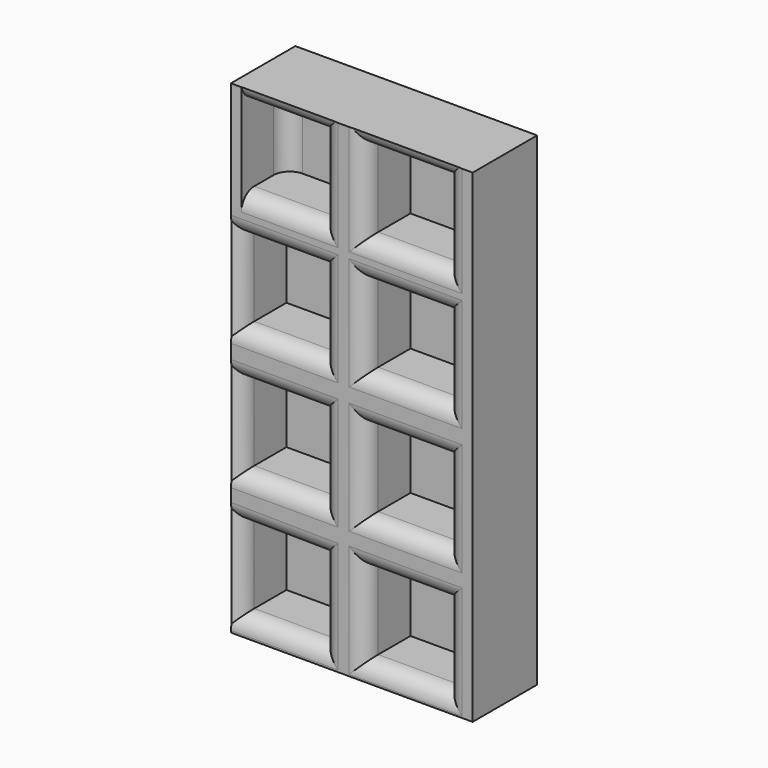
from build123d import *

# Parameters (mm, degrees)
F0_W          = 76.2
F0_H          = 152.4
F0_W_2        = 25.4
F0_H_2        = 25.4
F1_DEPTH      = 25.4
F2_DEPTH      = 7.62
F3_T1_DEPTH   = 25.4
F3_T3_DEPTH   = 25.4
F3_T5_DEPTH   = 25.4
F3_T7_DEPTH   = 25.4
F3_T9_DEPTH   = 25.4
F3_T11_DEPTH  = 25.4
F3_T13_DEPTH  = 25.4
F3_T18_DEPTH  = 50.8
F3_T23_DEPTH  = 50.8
F3_T28_DEPTH  = 50.8
F3_T33_DEPTH  = 50.8
F3_T38_DEPTH  = 50.8
F3_T43_DEPTH  = 50.8018343203
F3_T49_DEPTH  = 37.7319167972
F3_T54_DEPTH  = 38.0371819854
F3_T59_DEPTH  = 50.8
F3_T65_DEPTH  = 38.1
F3_T71_DEPTH  = 38.1
F3_T79_DEPTH  = 38.1
F3_T84_DEPTH  = 38.1
F3_T92_DEPTH  = 38.1
F3_T97_DEPTH  = 38.1
F3_T105_DEPTH = 38.1
F3_T110_DEPTH = 38.1
F3_T117_DEPTH = 38.1
F3_T122_DEPTH = 38.1
F3_T130_DEPTH = 38.1
F3_T135_DEPTH = 38.1
F3_T142_DEPTH = 38.1
F3_T147_DEPTH = 38.1
F3_T154_DEPTH = 38.1
F3_T158_DEPTH = 38.1
F3_T165_DEPTH = 38.1
F3_T171_DEPTH = 38.1
F3_T179_DEPTH = 38.1
F3_T184_DEPTH = 38.1
F3_T192_DEPTH = 38.1
F3_T197_DEPTH = 38.1
F3_T205_DEPTH = 38.1
F3_T209_DEPTH = 38.1
F3_T216_DEPTH = 38.1
F3_T220_DEPTH = 38.1
F3_T227_DEPTH = 38.1
F3_T232_DEPTH = 38.1
F3_T240_DEPTH = 38.1
F3_T244_DEPTH = 38.1
F3_T251_DEPTH = 38.1
F3_T255_DEPTH = 38.1
F3_T263_DEPTH = 38.1
F3_T267_DEPTH = 38.1
F3_T275_DEPTH = 38.1
F3_T279_DEPTH = 38.1
F3_T286_DEPTH = 38.1
F3_T290_DEPTH = 38.1
F3_T297_DEPTH = 38.1
F3_T302_DEPTH = 38.1
F3_T309_DEPTH = 38.1
F3_T314_DEPTH = 38.1
F3_T322_DEPTH = 38.1
F3_T326_DEPTH = 38.1
F3_T333_DEPTH = 38.1
F3_T338_DEPTH = 38.1
F3_T345_DEPTH = 38.1
F3_T350_DEPTH = 38.1
F3_T358_DEPTH = 38.1
F3_T362_DEPTH = 38.1
F3_T370_DEPTH = 38.0371819854
F3_T375_DEPTH = 50.8018343203
F3_T383_DEPTH = 50.8018343203
F3_T387_DEPTH = 37.7319167972
F3_T394_DEPTH = 38.1
F3_T398_DEPTH = 50.4319167972
F3_T406_DEPTH = 38.1
F3_T411_DEPTH = 50.7371819854
F3_T420_DEPTH = 38.1
F3_T425_DEPTH = 38.1


# Not quite as in the source:
# - a fillet or chamfer that OpenCascade refuses, or shapes differently, is made with other operations: its cross-section is extruded or revolved along the edge and cut away or added


with BuildPart() as f1:
    # F0 (on Front) → F1 (new body)
    with BuildSketch(Plane.XZ):
        Rectangle(F0_W, F0_H)
        Polygon((-34.8004736006, -70.5167502165), (-34.8004736006, -45.1795682311), (-9.4004736006, -45.4848334193), (-9.4004736006, -70.5167502165), align=None, mode=Mode.SUBTRACT)
        with Locations((-22.1004736006, -18.1948120378)):
            Rectangle(F0_W_2, F0_H_2, mode=Mode.SUBTRACT)
        with Locations((16.9737452313, -57.8795682311)):
            Rectangle(F0_W_2, F0_H_2, mode=Mode.SUBTRACT)
        with Locations((16.9737452313, -18.1948120378)):
            Rectangle(F0_W_2, F0_H_2, mode=Mode.SUBTRACT)
        with Locations((-22.1004736006, 21.8580199078)):
            Rectangle(F0_W_2, F0_H_2, mode=Mode.SUBTRACT)
        with Locations((-22.1004736006, 59.3430910587)):
            Rectangle(F0_W_2, F0_H_2, mode=Mode.SUBTRACT)
        with Locations((16.9737452313, 21.8580199078)):
            Rectangle(F0_W_2, F0_H_2, mode=Mode.SUBTRACT)
        with Locations((16.9737452313, 59.3430910587)):
            Rectangle(F0_W_2, F0_H_2, mode=Mode.SUBTRACT)
    extrude(amount=F1_DEPTH)

    # F0 (on Front) → F2 (join)
    with BuildSketch(Plane.XZ):
        with Locations((-22.1004736006, 59.3430910587)):
            Rectangle(F0_W_2, F0_H_2)
        with Locations((16.9737452313, 59.3430910587)):
            Rectangle(F0_W_2, F0_H_2)
        with Locations((16.9737452313, 21.8580199078)):
            Rectangle(F0_W_2, F0_H_2)
        with Locations((-22.1004736006, 21.8580199078)):
            Rectangle(F0_W_2, F0_H_2)
        with Locations((-22.1004736006, -18.1948120378)):
            Rectangle(F0_W_2, F0_H_2)
        with Locations((16.9737452313, -18.1948120378)):
            Rectangle(F0_W_2, F0_H_2)
        with Locations((16.9737452313, -57.8795682311)):
            Rectangle(F0_W_2, F0_H_2)
        Polygon((-9.4004736006, -45.4848334193), (-34.8004736006, -45.1795682311), (-34.8004736006, -70.5167502165), (-9.4004736006, -70.5167502165), align=None)
    extrude(amount=F2_DEPTH)

    # F3: fillet of radius 5.08 on 32 edges, made by hand

    # F3_s2 → F3_t1 (join)
    with BuildSketch(Plane.XY.offset(46.6430910587)):
        with BuildLine():
            ThreePointArc((-34.8004736006, -12.7), (-33.3125760491, -9.1078975516), (-29.7204736006, -7.62))
            Line((-29.7204736006, -7.62), (-34.8004736006, -7.62))
            Line((-34.8004736006, -7.62), (-34.8004736006, -12.7))
        make_face()
    extrude(amount=F3_T1_DEPTH)

    # F3_s4 → F3_t3 (cut)
    with BuildSketch(Plane.XY.offset(46.6430910587)):
        with BuildLine():
            ThreePointArc((34.7537452313, -25.4), (31.1616427829, -23.9121024484), (29.6737452313, -20.32))
            Line((29.6737452313, -20.32), (29.6737452313, -25.4))
            Line((29.6737452313, -25.4), (34.7537452313, -25.4))
        make_face()
        with BuildLine():
            ThreePointArc((-0.8062547687, -25.4), (2.7858476798, -23.9121024484), (4.2737452313, -20.32))
            Line((4.2737452313, -20.32), (4.2737452313, -25.4))
            Line((4.2737452313, -25.4), (-0.8062547687, -25.4))
        make_face()
        with BuildLine():
            ThreePointArc((-4.3204736006, -25.4), (-7.9125760491, -23.9121024484), (-9.4004736006, -20.32))
            Line((-9.4004736006, -20.32), (-9.4004736006, -25.4))
            Line((-9.4004736006, -25.4), (-4.3204736006, -25.4))
        make_face()
    extrude(amount=F3_T3_DEPTH, mode=Mode.SUBTRACT)

    # F3_s6 → F3_t5 (cut)
    with BuildSketch(Plane.YZ.offset(4.2737452313)):
        with BuildLine():
            ThreePointArc((-25.4, 77.1230910587), (-23.9121024484, 73.5309886103), (-20.32, 72.0430910587))
            Line((-20.32, 72.0430910587), (-25.4, 72.0430910587))
            Line((-25.4, 72.0430910587), (-25.4, 77.1230910587))
        make_face()
        with BuildLine():
            ThreePointArc((-25.4, 41.5630910587), (-23.9121024484, 45.1551935072), (-20.32, 46.6430910587))
            Line((-20.32, 46.6430910587), (-25.4, 46.6430910587))
            Line((-25.4, 46.6430910587), (-25.4, 41.5630910587))
        make_face()
        with BuildLine():
            ThreePointArc((-25.4, -0.4148120378), (-23.9121024484, -4.0069144862), (-20.32, -5.4948120378))
            Line((-20.32, -5.4948120378), (-25.4, -5.4948120378))
            Line((-25.4, -5.4948120378), (-25.4, -0.4148120378))
        make_face()
        with BuildLine():
            ThreePointArc((-25.4, -35.9748120378), (-23.9121024484, -32.3827095894), (-20.32, -30.8948120378))
            Line((-20.32, -30.8948120378), (-25.4, -30.8948120378))
            Line((-25.4, -30.8948120378), (-25.4, -35.9748120378))
        make_face()
        with BuildLine():
            ThreePointArc((-25.4, 39.6380199078), (-23.9121024484, 36.0459174593), (-20.32, 34.5580199078))
            Line((-20.32, 34.5580199078), (-25.4, 34.5580199078))
            Line((-25.4, 34.5580199078), (-25.4, 39.6380199078))
        make_face()
        with BuildLine():
            ThreePointArc((-25.4, -40.0995682311), (-23.9121024484, -43.6916706795), (-20.32, -45.1795682311))
            Line((-20.32, -45.1795682311), (-25.4, -45.1795682311))
            Line((-25.4, -45.1795682311), (-25.4, -40.0995682311))
        make_face()
        with BuildLine():
            ThreePointArc((-25.4, -75.6595682311), (-23.9121024484, -72.0674657827), (-20.32, -70.5795682311))
            Line((-20.32, -70.5795682311), (-25.4, -70.5795682311))
            Line((-25.4, -70.5795682311), (-25.4, -75.6595682311))
        make_face()
        with BuildLine():
            ThreePointArc((-25.4, 4.0780199078), (-23.9121024484, 7.6701223562), (-20.32, 9.1580199078))
            Line((-20.32, 9.1580199078), (-25.4, 9.1580199078))
            Line((-25.4, 9.1580199078), (-25.4, 4.0780199078))
        make_face()
    extrude(amount=F3_T5_DEPTH, mode=Mode.SUBTRACT)

    # F3_s8 → F3_t7 (cut)
    with BuildSketch(Plane.YZ.offset(-34.8004736006)):
        with BuildLine():
            ThreePointArc((-25.4, 77.1230910587), (-23.9121024484, 73.5309886103), (-20.32, 72.0430910587))
            Line((-20.32, 72.0430910587), (-25.4, 72.0430910587))
            Line((-25.4, 72.0430910587), (-25.4, 77.1230910587))
        make_face()
        with BuildLine():
            ThreePointArc((-25.4, 41.5630910587), (-23.9121024484, 45.1551935072), (-20.32, 46.6430910587))
            Line((-20.32, 46.6430910587), (-25.4, 46.6430910587))
            Line((-25.4, 46.6430910587), (-25.4, 41.5630910587))
        make_face()
        with BuildLine():
            ThreePointArc((-25.4, 39.6380199078), (-23.9121024484, 36.0459174593), (-20.32, 34.5580199078))
            Line((-20.32, 34.5580199078), (-25.4, 34.5580199078))
            Line((-25.4, 34.5580199078), (-25.4, 39.6380199078))
        make_face()
        with BuildLine():
            ThreePointArc((-25.4, 4.0780199078), (-23.9121024484, 7.6701223562), (-20.32, 9.1580199078))
            Line((-20.32, 9.1580199078), (-25.4, 9.1580199078))
            Line((-25.4, 9.1580199078), (-25.4, 4.0780199078))
        make_face()
        with BuildLine():
            ThreePointArc((-25.4, -0.4148120378), (-23.9121024484, -4.0069144862), (-20.32, -5.4948120378))
            Line((-20.32, -5.4948120378), (-25.4, -5.4948120378))
            Line((-25.4, -5.4948120378), (-25.4, -0.4148120378))
        make_face()
        with BuildLine():
            ThreePointArc((-25.4, -35.9748120378), (-23.9121024484, -32.3827095894), (-20.32, -30.8948120378))
            Line((-20.32, -30.8948120378), (-25.4, -30.8948120378))
            Line((-25.4, -30.8948120378), (-25.4, -35.9748120378))
        make_face()
        with BuildLine():
            ThreePointArc((-25.4, -75.5967502165), (-23.9121024484, -72.0046477681), (-20.32, -70.5167502165))
            Line((-20.32, -70.5167502165), (-25.4, -70.5167502165))
            Line((-25.4, -70.5167502165), (-25.4, -75.5967502165))
        make_face()
    extrude(amount=F3_T7_DEPTH, mode=Mode.SUBTRACT)

    # F3_s10 → F3_t9 (cut)
    with BuildSketch(Plane.XY.offset(9.1580199078)):
        with BuildLine():
            ThreePointArc((-4.3204736006, -25.4), (-7.9125760491, -23.9121024484), (-9.4004736006, -20.32))
            Line((-9.4004736006, -20.32), (-9.4004736006, -25.4))
            Line((-9.4004736006, -25.4), (-4.3204736006, -25.4))
        make_face()
        with BuildLine():
            ThreePointArc((-39.8804736006, -25.4), (-36.2883711522, -23.9121024484), (-34.8004736006, -20.32))
            Line((-34.8004736006, -20.32), (-34.8004736006, -25.4))
            Line((-34.8004736006, -25.4), (-39.8804736006, -25.4))
        make_face()
        with BuildLine():
            ThreePointArc((-0.8062547687, -25.4), (2.7858476798, -23.9121024484), (4.2737452313, -20.32))
            Line((4.2737452313, -20.32), (4.2737452313, -25.4))
            Line((4.2737452313, -25.4), (-0.8062547687, -25.4))
        make_face()
        with BuildLine():
            ThreePointArc((34.7537452313, -25.4), (31.1616427829, -23.9121024484), (29.6737452313, -20.32))
            Line((29.6737452313, -20.32), (29.6737452313, -25.4))
            Line((29.6737452313, -25.4), (34.7537452313, -25.4))
        make_face()
    extrude(amount=F3_T9_DEPTH, mode=Mode.SUBTRACT)

    # F3_s12 → F3_t11 (cut)
    with BuildSketch(Plane.XY.offset(-30.8948120378)):
        with BuildLine():
            ThreePointArc((-4.3204736006, -25.4), (-7.9125760491, -23.9121024484), (-9.4004736006, -20.32))
            Line((-9.4004736006, -20.32), (-9.4004736006, -25.4))
            Line((-9.4004736006, -25.4), (-4.3204736006, -25.4))
        make_face()
        with BuildLine():
            ThreePointArc((-39.8804736006, -25.4), (-36.2883711522, -23.9121024484), (-34.8004736006, -20.32))
            Line((-34.8004736006, -20.32), (-34.8004736006, -25.4))
            Line((-34.8004736006, -25.4), (-39.8804736006, -25.4))
        make_face()
        with BuildLine():
            ThreePointArc((34.7537452313, -25.4), (31.1616427829, -23.9121024484), (29.6737452313, -20.32))
            Line((29.6737452313, -20.32), (29.6737452313, -25.4))
            Line((29.6737452313, -25.4), (34.7537452313, -25.4))
        make_face()
        with BuildLine():
            ThreePointArc((-0.8062547687, -25.4), (2.7858476798, -23.9121024484), (4.2737452313, -20.32))
            Line((4.2737452313, -20.32), (4.2737452313, -25.4))
            Line((4.2737452313, -25.4), (-0.8062547687, -25.4))
        make_face()
    extrude(amount=F3_T11_DEPTH, mode=Mode.SUBTRACT)

    # F3_s14 → F3_t13 (cut)
    with BuildSketch(Plane.XY.offset(-70.5795682311)):
        with BuildLine():
            ThreePointArc((34.7537452313, -25.4), (31.1616427829, -23.9121024484), (29.6737452313, -20.32))
            Line((29.6737452313, -20.32), (29.6737452313, -25.4))
            Line((29.6737452313, -25.4), (34.7537452313, -25.4))
        make_face()
        with BuildLine():
            ThreePointArc((-0.8062547687, -25.4), (2.7858476798, -23.9121024484), (4.2737452313, -20.32))
            Line((4.2737452313, -20.32), (4.2737452313, -25.4))
            Line((4.2737452313, -25.4), (-0.8062547687, -25.4))
        make_face()
    extrude(amount=F3_T13_DEPTH, mode=Mode.SUBTRACT)


with BuildPart() as f3_tool16:
    # F3_s17 → F3_t18 (new body)
    with BuildSketch(Plane.XY.offset(84.7430910587)):
        with BuildLine():
            ThreePointArc((34.7537452313, -25.4), (31.1616427829, -23.9121024484), (29.6737452313, -20.32))
            Line((29.6737452313, -20.32), (29.6737452313, -25.4))
            Line((29.6737452313, -25.4), (34.7537452313, -25.4))
        make_face()
    extrude(amount=-F3_T18_DEPTH)

    split(bisect_by=Plane.XY.offset(34.5580199078), keep=Keep.BOTTOM)


with BuildPart() as f1_1:
    add(f1.part)

    # F3_t15: cut F3_tool16
    add(f3_tool16.part, mode=Mode.SUBTRACT)


with BuildPart() as f3_tool21:
    # F3_s22 → F3_t23 (new body)
    with BuildSketch(Plane.XY.offset(33.9430910587)):
        with BuildLine():
            ThreePointArc((-0.8062547687, -25.4), (2.7858476798, -23.9121024484), (4.2737452313, -20.32))
            Line((4.2737452313, -20.32), (4.2737452313, -25.4))
            Line((4.2737452313, -25.4), (-0.8062547687, -25.4))
        make_face()
    extrude(amount=F3_T23_DEPTH)

    split(bisect_by=Plane.XY.offset(34.5580199078), keep=Keep.BOTTOM)


with BuildPart() as f1_2:
    add(f1_1.part)

    # F3_t20: cut F3_tool21
    add(f3_tool21.part, mode=Mode.SUBTRACT)


with BuildPart() as f3_tool26:
    # F3_s27 → F3_t28 (new body)
    with BuildSketch(Plane.XY.offset(84.7430910587)):
        with BuildLine():
            ThreePointArc((-4.3204736006, -25.4), (-7.9125760491, -23.9121024484), (-9.4004736006, -20.32))
            Line((-9.4004736006, -20.32), (-9.4004736006, -25.4))
            Line((-9.4004736006, -25.4), (-4.3204736006, -25.4))
        make_face()
    extrude(amount=-F3_T28_DEPTH)

    split(bisect_by=Plane.XY.offset(34.5580199078), keep=Keep.BOTTOM)


with BuildPart() as f1_3:
    add(f1_2.part)

    # F3_t25: cut F3_tool26
    add(f3_tool26.part, mode=Mode.SUBTRACT)


with BuildPart() as f3_tool31:
    # F3_s32 → F3_t33 (new body)
    with BuildSketch(Plane.XY.offset(47.2580199078)):
        with BuildLine():
            ThreePointArc((-4.3204736006, -25.4), (-7.9125760491, -23.9121024484), (-9.4004736006, -20.32))
            Line((-9.4004736006, -20.32), (-9.4004736006, -25.4))
            Line((-9.4004736006, -25.4), (-4.3204736006, -25.4))
        make_face()
    extrude(amount=-F3_T33_DEPTH)

    split(bisect_by=Plane.XY.offset(46.6430910587), keep=Keep.TOP)


with BuildPart() as f1_4:
    add(f1_3.part)

    # F3_t30: cut F3_tool31
    add(f3_tool31.part, mode=Mode.SUBTRACT)


with BuildPart() as f3_tool36:
    # F3_s37 → F3_t38 (new body)
    with BuildSketch(Plane.XY.offset(-3.5419800922)):
        with BuildLine():
            ThreePointArc((-0.8062547687, -25.4), (2.7858476798, -23.9121024484), (4.2737452313, -20.32))
            Line((4.2737452313, -20.32), (4.2737452313, -25.4))
            Line((4.2737452313, -25.4), (-0.8062547687, -25.4))
        make_face()
    extrude(amount=F3_T38_DEPTH)

    split(bisect_by=Plane.XY.offset(46.6430910587), keep=Keep.TOP)


with BuildPart() as f1_5:
    add(f1_4.part)

    # F3_t35: cut F3_tool36
    add(f3_tool36.part, mode=Mode.SUBTRACT)


with BuildPart() as f3_tool41:
    # F3_s42 → F3_t43 (new body)
    with BuildSketch(Plane(origin=(-46.9516268134, 0, 0.5642794172), x_dir=(0, 1, 0), z_dir=(0.9999277879, 0, -0.0120174466))):
        with BuildLine():
            ThreePointArc((-25.4, -40.5145185529), (-23.9121024484, -44.1066210013), (-20.32, -45.5945185529))
            Line((-20.32, -45.5945185529), (-25.4, -45.5945185529))
            Line((-25.4, -45.5945185529), (-25.4, -40.5145185529))
        make_face()
    extrude(amount=F3_T43_DEPTH)

    split(bisect_by=Plane.YZ.offset(-34.8004736006), keep=Keep.TOP)

    split(bisect_by=Plane.YZ.offset(-9.4004736006), keep=Keep.BOTTOM)


with BuildPart() as f1_6:
    add(f1_5.part)

    # F3_t40: cut F3_tool41
    add(f3_tool41.part, mode=Mode.SUBTRACT)


with BuildPart() as f3_tool47:
    # F3_s48 → F3_t49 (new body)
    with BuildSketch(Plane.XY.offset(-32.7848334193)):
        with BuildLine():
            ThreePointArc((-4.3204736006, -25.4), (-7.9125760491, -23.9121024484), (-9.4004736006, -20.32))
            Line((-9.4004736006, -20.32), (-9.4004736006, -25.4))
            Line((-9.4004736006, -25.4), (-4.3204736006, -25.4))
        make_face()
    extrude(amount=-F3_T49_DEPTH)

    split(bisect_by=Plane(origin=(-0.5479296933, 0, -45.5912260761), x_dir=(0, 1, 0), z_dir=(-0.0120174466, 0, -0.9999277879)), keep=Keep.TOP)


with BuildPart() as f1_7:
    add(f1_6.part)

    # F3_t46: cut F3_tool47
    add(f3_tool47.part, mode=Mode.SUBTRACT)


with BuildPart() as f3_tool52:
    # F3_s53 → F3_t54 (new body)
    with BuildSketch(Plane.XY.offset(-70.5167502165)):
        with BuildLine():
            ThreePointArc((-39.8804736006, -25.4), (-36.2883711522, -23.9121024484), (-34.8004736006, -20.32))
            Line((-34.8004736006, -20.32), (-34.8004736006, -25.4))
            Line((-34.8004736006, -25.4), (-39.8804736006, -25.4))
        make_face()
    extrude(amount=F3_T54_DEPTH)

    split(bisect_by=Plane(origin=(-0.5479296933, 0, -45.5912260761), x_dir=(0, 1, 0), z_dir=(-0.0120174466, 0, -0.9999277879)), keep=Keep.TOP)


with BuildPart() as f1_8:
    add(f1_7.part)

    # F3_t51: cut F3_tool52
    add(f3_tool52.part, mode=Mode.SUBTRACT)


with BuildPart() as f3_tool57:
    # F3_s58 → F3_t59 (new body)
    with BuildSketch(Plane.XY.offset(47.2580199078)):
        with BuildLine():
            ThreePointArc((34.7537452313, -25.4), (31.1616427829, -23.9121024484), (29.6737452313, -20.32))
            Line((29.6737452313, -20.32), (29.6737452313, -25.4))
            Line((29.6737452313, -25.4), (34.7537452313, -25.4))
        make_face()
    extrude(amount=-F3_T59_DEPTH)

    split(bisect_by=Plane.XY.offset(46.6430910587), keep=Keep.TOP)


with BuildPart() as f1_9:
    add(f1_8.part)

    # F3_t56: cut F3_tool57
    add(f3_tool57.part, mode=Mode.SUBTRACT)


with BuildPart() as f3_tool63:
    # F3_s64 → F3_t65 (new body)
    with BuildSketch(Plane.YZ.offset(4.2737452313)):
        with BuildLine():
            ThreePointArc((-25.4, 77.1230910587), (-23.9121024484, 73.5309886103), (-20.32, 72.0430910587))
            Line((-20.32, 72.0430910587), (-25.4, 72.0430910587))
            Line((-25.4, 72.0430910587), (-25.4, 77.1230910587))
        make_face()
    extrude(amount=F3_T65_DEPTH)

    split(bisect_by=Plane.YZ.offset(38.1), keep=Keep.BOTTOM)

    split(bisect_by=Plane.XY.offset(76.2), keep=Keep.BOTTOM)

    split(bisect_by=Plane.YZ.offset(29.6737452313), keep=Keep.TOP)


with BuildPart() as f3_tool69:
    # F3_s70 → F3_t71 (new body)
    with BuildSketch(Plane.XY.offset(84.7430910587)):
        with BuildLine():
            ThreePointArc((34.7537452313, -25.4), (31.1616427829, -23.9121024484), (29.6737452313, -20.32))
            Line((29.6737452313, -20.32), (29.6737452313, -25.4))
            Line((29.6737452313, -25.4), (34.7537452313, -25.4))
        make_face()
    extrude(amount=-F3_T71_DEPTH)

    split(bisect_by=Plane.XY.offset(76.2), keep=Keep.BOTTOM)

    split(bisect_by=Plane.XY.offset(72.0430910587), keep=Keep.TOP)


with BuildPart() as f3_tool63_1:
    add(f3_tool63.part)

    # F3_t74: intersect F3_tool69
    add(f3_tool69.part, mode=Mode.INTERSECT)


with BuildPart() as f1_10:
    add(f1_9.part)

    # F3_t61: cut F3_tool63
    add(f3_tool63_1.part, mode=Mode.SUBTRACT)


with BuildPart() as f3_tool77:
    # F3_s78 → F3_t79 (new body)
    with BuildSketch(Plane.XY.offset(72.0430910587)):
        with BuildLine():
            ThreePointArc((34.7537452313, -25.4), (31.1616427829, -23.9121024484), (29.6737452313, -20.32))
            Line((29.6737452313, -20.32), (29.6737452313, -25.4))
            Line((29.6737452313, -25.4), (34.7537452313, -25.4))
        make_face()
    extrude(amount=-F3_T79_DEPTH)

    split(bisect_by=Plane.XY.offset(34.5580199078), keep=Keep.TOP)

    split(bisect_by=Plane.XY.offset(46.6430910587), keep=Keep.BOTTOM)


with BuildPart() as f3_tool82:
    # F3_s83 → F3_t84 (new body)
    with BuildSketch(Plane.YZ.offset(42.3737452313)):
        with BuildLine():
            ThreePointArc((-25.4, 41.5630910587), (-23.9121024484, 45.1551935072), (-20.32, 46.6430910587))
            Line((-20.32, 46.6430910587), (-25.4, 46.6430910587))
            Line((-25.4, 46.6430910587), (-25.4, 41.5630910587))
        make_face()
    extrude(amount=-F3_T84_DEPTH)

    split(bisect_by=Plane.YZ.offset(38.1), keep=Keep.BOTTOM)

    split(bisect_by=Plane.YZ.offset(29.6737452313), keep=Keep.TOP)


with BuildPart() as f3_tool77_1:
    add(f3_tool77.part)

    # F3_t87: intersect F3_tool82
    add(f3_tool82.part, mode=Mode.INTERSECT)


with BuildPart() as f1_11:
    add(f1_10.part)

    # F3_t75: cut F3_tool77
    add(f3_tool77_1.part, mode=Mode.SUBTRACT)


with BuildPart() as f3_tool90:
    # F3_s91 → F3_t92 (new body)
    with BuildSketch(Plane.XY.offset(46.6430910587)):
        with BuildLine():
            ThreePointArc((-0.8062547687, -25.4), (2.7858476798, -23.9121024484), (4.2737452313, -20.32))
            Line((4.2737452313, -20.32), (4.2737452313, -25.4))
            Line((4.2737452313, -25.4), (-0.8062547687, -25.4))
        make_face()
    extrude(amount=F3_T92_DEPTH)

    split(bisect_by=Plane.XY.offset(76.2), keep=Keep.BOTTOM)

    split(bisect_by=Plane.XY.offset(72.0430910587), keep=Keep.TOP)


with BuildPart() as f3_tool95:
    # F3_s96 → F3_t97 (new body)
    with BuildSketch(Plane.YZ.offset(-8.4262547687)):
        with BuildLine():
            ThreePointArc((-25.4, 77.1230910587), (-23.9121024484, 73.5309886103), (-20.32, 72.0430910587))
            Line((-20.32, 72.0430910587), (-25.4, 72.0430910587))
            Line((-25.4, 72.0430910587), (-25.4, 77.1230910587))
        make_face()
    extrude(amount=F3_T97_DEPTH)

    split(bisect_by=Plane.XY.offset(76.2), keep=Keep.BOTTOM)

    split(bisect_by=Plane.YZ.offset(4.2737452313), keep=Keep.BOTTOM)


with BuildPart() as f3_tool90_1:
    add(f3_tool90.part)

    # F3_t100: intersect F3_tool95
    add(f3_tool95.part, mode=Mode.INTERSECT)


with BuildPart() as f1_12:
    add(f1_11.part)

    # F3_t88: cut F3_tool90
    add(f3_tool90_1.part, mode=Mode.SUBTRACT)


with BuildPart() as f3_tool103:
    # F3_s104 → F3_t105 (new body)
    with BuildSketch(Plane.XY.offset(33.9430910587)):
        with BuildLine():
            ThreePointArc((-0.8062547687, -25.4), (2.7858476798, -23.9121024484), (4.2737452313, -20.32))
            Line((4.2737452313, -20.32), (4.2737452313, -25.4))
            Line((4.2737452313, -25.4), (-0.8062547687, -25.4))
        make_face()
    extrude(amount=F3_T105_DEPTH)

    split(bisect_by=Plane.XY.offset(34.5580199078), keep=Keep.TOP)

    split(bisect_by=Plane.XY.offset(46.6430910587), keep=Keep.BOTTOM)


with BuildPart() as f3_tool108:
    # F3_s109 → F3_t110 (new body)
    with BuildSketch(Plane.YZ.offset(29.6737452313)):
        with BuildLine():
            ThreePointArc((-25.4, 41.5630910587), (-23.9121024484, 45.1551935072), (-20.32, 46.6430910587))
            Line((-20.32, 46.6430910587), (-25.4, 46.6430910587))
            Line((-25.4, 46.6430910587), (-25.4, 41.5630910587))
        make_face()
    extrude(amount=-F3_T110_DEPTH)

    split(bisect_by=Plane.YZ.offset(4.2737452313), keep=Keep.BOTTOM)


with BuildPart() as f3_tool103_1:
    add(f3_tool103.part)

    # F3_t112: intersect F3_tool108
    add(f3_tool108.part, mode=Mode.INTERSECT)


with BuildPart() as f1_13:
    add(f1_12.part)

    # F3_t101: cut F3_tool103
    add(f3_tool103_1.part, mode=Mode.SUBTRACT)


with BuildPart() as f3_tool115:
    # F3_s116 → F3_t117 (new body)
    with BuildSketch(Plane.YZ.offset(-34.8004736006)):
        with BuildLine():
            ThreePointArc((-25.4, 77.1230910587), (-23.9121024484, 73.5309886103), (-20.32, 72.0430910587))
            Line((-20.32, 72.0430910587), (-25.4, 72.0430910587))
            Line((-25.4, 72.0430910587), (-25.4, 77.1230910587))
        make_face()
    extrude(amount=F3_T117_DEPTH)

    split(bisect_by=Plane.XY.offset(76.2), keep=Keep.BOTTOM)

    split(bisect_by=Plane.YZ.offset(-9.4004736006), keep=Keep.TOP)


with BuildPart() as f3_tool120:
    # F3_s121 → F3_t122 (new body)
    with BuildSketch(Plane.XY.offset(84.7430910587)):
        with BuildLine():
            ThreePointArc((-4.3204736006, -25.4), (-7.9125760491, -23.9121024484), (-9.4004736006, -20.32))
            Line((-9.4004736006, -20.32), (-9.4004736006, -25.4))
            Line((-9.4004736006, -25.4), (-4.3204736006, -25.4))
        make_face()
    extrude(amount=-F3_T122_DEPTH)

    split(bisect_by=Plane.XY.offset(76.2), keep=Keep.BOTTOM)

    split(bisect_by=Plane.XY.offset(72.0430910587), keep=Keep.TOP)


with BuildPart() as f3_tool115_1:
    add(f3_tool115.part)

    # F3_t125: intersect F3_tool120
    add(f3_tool120.part, mode=Mode.INTERSECT)


with BuildPart() as f1_14:
    add(f1_13.part)

    # F3_t113: cut F3_tool115
    add(f3_tool115_1.part, mode=Mode.SUBTRACT)


with BuildPart() as f3_tool128:
    # F3_s129 → F3_t130 (new body)
    with BuildSketch(Plane.XY.offset(72.0430910587)):
        with BuildLine():
            ThreePointArc((-4.3204736006, -25.4), (-7.9125760491, -23.9121024484), (-9.4004736006, -20.32))
            Line((-9.4004736006, -20.32), (-9.4004736006, -25.4))
            Line((-9.4004736006, -25.4), (-4.3204736006, -25.4))
        make_face()
    extrude(amount=-F3_T130_DEPTH)

    split(bisect_by=Plane.XY.offset(34.5580199078), keep=Keep.TOP)

    split(bisect_by=Plane.XY.offset(46.6430910587), keep=Keep.BOTTOM)


with BuildPart() as f3_tool133:
    # F3_s134 → F3_t135 (new body)
    with BuildSketch(Plane.YZ.offset(3.2995263994)):
        with BuildLine():
            ThreePointArc((-25.4, 41.5630910587), (-23.9121024484, 45.1551935072), (-20.32, 46.6430910587))
            Line((-20.32, 46.6430910587), (-25.4, 46.6430910587))
            Line((-25.4, 46.6430910587), (-25.4, 41.5630910587))
        make_face()
    extrude(amount=-F3_T135_DEPTH)

    split(bisect_by=Plane.YZ.offset(-9.4004736006), keep=Keep.TOP)


with BuildPart() as f3_tool128_1:
    add(f3_tool128.part)

    # F3_t137: intersect F3_tool133
    add(f3_tool133.part, mode=Mode.INTERSECT)


with BuildPart() as f1_15:
    add(f1_14.part)

    # F3_t126: cut F3_tool128
    add(f3_tool128_1.part, mode=Mode.SUBTRACT)


with BuildPart() as f3_tool140:
    # F3_s141 → F3_t142 (new body)
    with BuildSketch(Plane.XY.offset(47.2580199078)):
        with BuildLine():
            ThreePointArc((-4.3204736006, -25.4), (-7.9125760491, -23.9121024484), (-9.4004736006, -20.32))
            Line((-9.4004736006, -20.32), (-9.4004736006, -25.4))
            Line((-9.4004736006, -25.4), (-4.3204736006, -25.4))
        make_face()
    extrude(amount=-F3_T142_DEPTH)

    split(bisect_by=Plane.XY.offset(34.5580199078), keep=Keep.TOP)

    split(bisect_by=Plane.XY.offset(46.6430910587), keep=Keep.BOTTOM)


with BuildPart() as f3_tool145:
    # F3_s146 → F3_t147 (new body)
    with BuildSketch(Plane.YZ.offset(-34.8004736006)):
        with BuildLine():
            ThreePointArc((-25.4, 39.6380199078), (-23.9121024484, 36.0459174593), (-20.32, 34.5580199078))
            Line((-20.32, 34.5580199078), (-25.4, 34.5580199078))
            Line((-25.4, 34.5580199078), (-25.4, 39.6380199078))
        make_face()
    extrude(amount=F3_T147_DEPTH)

    split(bisect_by=Plane.YZ.offset(-9.4004736006), keep=Keep.TOP)


with BuildPart() as f3_tool140_1:
    add(f3_tool140.part)

    # F3_t149: intersect F3_tool145
    add(f3_tool145.part, mode=Mode.INTERSECT)


with BuildPart() as f1_16:
    add(f1_15.part)

    # F3_t138: cut F3_tool140
    add(f3_tool140_1.part, mode=Mode.SUBTRACT)


with BuildPart() as f3_tool152:
    # F3_s153 → F3_t154 (new body)
    with BuildSketch(Plane.XY.offset(34.5580199078)):
        with BuildLine():
            ThreePointArc((-4.3204736006, -25.4), (-7.9125760491, -23.9121024484), (-9.4004736006, -20.32))
            Line((-9.4004736006, -20.32), (-9.4004736006, -25.4))
            Line((-9.4004736006, -25.4), (-4.3204736006, -25.4))
        make_face()
    extrude(amount=-F3_T154_DEPTH)

    split(bisect_by=Plane.XY.offset(9.1580199078), keep=Keep.BOTTOM)


with BuildPart() as f3_tool156:
    # F3_s157 → F3_t158 (new body)
    with BuildSketch(Plane.YZ.offset(3.2995263994)):
        with BuildLine():
            ThreePointArc((-25.4, 4.0780199078), (-23.9121024484, 7.6701223562), (-20.32, 9.1580199078))
            Line((-20.32, 9.1580199078), (-25.4, 9.1580199078))
            Line((-25.4, 9.1580199078), (-25.4, 4.0780199078))
        make_face()
    extrude(amount=-F3_T158_DEPTH)

    split(bisect_by=Plane.YZ.offset(-9.4004736006), keep=Keep.TOP)


with BuildPart() as f3_tool152_1:
    add(f3_tool152.part)

    # F3_t160: intersect F3_tool156
    add(f3_tool156.part, mode=Mode.INTERSECT)


with BuildPart() as f1_17:
    add(f1_16.part)

    # F3_t150: cut F3_tool152
    add(f3_tool152_1.part, mode=Mode.SUBTRACT)


with BuildPart() as f3_tool163:
    # F3_s164 → F3_t165 (new body)
    with BuildSketch(Plane.XY.offset(9.1580199078)):
        with BuildLine():
            ThreePointArc((-39.8804736006, -25.4), (-36.2883711522, -23.9121024484), (-34.8004736006, -20.32))
            Line((-34.8004736006, -20.32), (-34.8004736006, -25.4))
            Line((-34.8004736006, -25.4), (-39.8804736006, -25.4))
        make_face()
    extrude(amount=F3_T165_DEPTH)

    split(bisect_by=Plane.YZ.offset(-38.1), keep=Keep.TOP)

    split(bisect_by=Plane.XY.offset(34.5580199078), keep=Keep.TOP)

    split(bisect_by=Plane.XY.offset(46.6430910587), keep=Keep.BOTTOM)


with BuildPart() as f3_tool169:
    # F3_s170 → F3_t171 (new body)
    with BuildSketch(Plane.YZ.offset(-47.5004736006)):
        with BuildLine():
            ThreePointArc((-25.4, 39.6380199078), (-23.9121024484, 36.0459174593), (-20.32, 34.5580199078))
            Line((-20.32, 34.5580199078), (-25.4, 34.5580199078))
            Line((-25.4, 34.5580199078), (-25.4, 39.6380199078))
        make_face()
    extrude(amount=F3_T171_DEPTH)

    split(bisect_by=Plane.YZ.offset(-38.1), keep=Keep.TOP)

    split(bisect_by=Plane.YZ.offset(-34.8004736006), keep=Keep.BOTTOM)


with BuildPart() as f3_tool163_1:
    add(f3_tool163.part)

    # F3_t174: intersect F3_tool169
    add(f3_tool169.part, mode=Mode.INTERSECT)


with BuildPart() as f1_18:
    add(f1_17.part)

    # F3_t161: cut F3_tool163
    add(f3_tool163_1.part, mode=Mode.SUBTRACT)


with BuildPart() as f3_tool177:
    # F3_s178 → F3_t179 (new body)
    with BuildSketch(Plane.YZ.offset(-9.4004736006)):
        with BuildLine():
            ThreePointArc((-25.4, 4.0780199078), (-23.9121024484, 7.6701223562), (-20.32, 9.1580199078))
            Line((-20.32, 9.1580199078), (-25.4, 9.1580199078))
            Line((-25.4, 9.1580199078), (-25.4, 4.0780199078))
        make_face()
    extrude(amount=-F3_T179_DEPTH)

    split(bisect_by=Plane.YZ.offset(-38.1), keep=Keep.TOP)

    split(bisect_by=Plane.YZ.offset(-34.8004736006), keep=Keep.BOTTOM)


with BuildPart() as f3_tool182:
    # F3_s183 → F3_t184 (new body)
    with BuildSketch(Plane.XY.offset(-3.5419800922)):
        with BuildLine():
            ThreePointArc((-39.8804736006, -25.4), (-36.2883711522, -23.9121024484), (-34.8004736006, -20.32))
            Line((-34.8004736006, -20.32), (-34.8004736006, -25.4))
            Line((-34.8004736006, -25.4), (-39.8804736006, -25.4))
        make_face()
    extrude(amount=F3_T184_DEPTH)

    split(bisect_by=Plane.YZ.offset(-38.1), keep=Keep.TOP)

    split(bisect_by=Plane.XY.offset(9.1580199078), keep=Keep.BOTTOM)


with BuildPart() as f3_tool177_1:
    add(f3_tool177.part)

    # F3_t187: intersect F3_tool182
    add(f3_tool182.part, mode=Mode.INTERSECT)


with BuildPart() as f1_19:
    add(f1_18.part)

    # F3_t175: cut F3_tool177
    add(f3_tool177_1.part, mode=Mode.SUBTRACT)


with BuildPart() as f3_tool190:
    # F3_s191 → F3_t192 (new body)
    with BuildSketch(Plane.XY.offset(-30.8948120378)):
        with BuildLine():
            ThreePointArc((-39.8804736006, -25.4), (-36.2883711522, -23.9121024484), (-34.8004736006, -20.32))
            Line((-34.8004736006, -20.32), (-34.8004736006, -25.4))
            Line((-34.8004736006, -25.4), (-39.8804736006, -25.4))
        make_face()
    extrude(amount=F3_T192_DEPTH)

    split(bisect_by=Plane.YZ.offset(-38.1), keep=Keep.TOP)

    split(bisect_by=Plane.XY.offset(-5.4948120378), keep=Keep.TOP)


with BuildPart() as f3_tool195:
    # F3_s196 → F3_t197 (new body)
    with BuildSketch(Plane.YZ.offset(-47.5004736006)):
        with BuildLine():
            ThreePointArc((-25.4, -0.4148120378), (-23.9121024484, -4.0069144862), (-20.32, -5.4948120378))
            Line((-20.32, -5.4948120378), (-25.4, -5.4948120378))
            Line((-25.4, -5.4948120378), (-25.4, -0.4148120378))
        make_face()
    extrude(amount=F3_T197_DEPTH)

    split(bisect_by=Plane.YZ.offset(-38.1), keep=Keep.TOP)

    split(bisect_by=Plane.YZ.offset(-34.8004736006), keep=Keep.BOTTOM)


with BuildPart() as f3_tool190_1:
    add(f3_tool190.part)

    # F3_t200: intersect F3_tool195
    add(f3_tool195.part, mode=Mode.INTERSECT)


with BuildPart() as f1_20:
    add(f1_19.part)

    # F3_t188: cut F3_tool190
    add(f3_tool190_1.part, mode=Mode.SUBTRACT)


with BuildPart() as f3_tool203:
    # F3_s204 → F3_t205 (new body)
    with BuildSketch(Plane.YZ.offset(-34.8004736006)):
        with BuildLine():
            ThreePointArc((-25.4, -0.4148120378), (-23.9121024484, -4.0069144862), (-20.32, -5.4948120378))
            Line((-20.32, -5.4948120378), (-25.4, -5.4948120378))
            Line((-25.4, -5.4948120378), (-25.4, -0.4148120378))
        make_face()
    extrude(amount=F3_T205_DEPTH)

    split(bisect_by=Plane.YZ.offset(-9.4004736006), keep=Keep.TOP)


with BuildPart() as f3_tool207:
    # F3_s208 → F3_t209 (new body)
    with BuildSketch(Plane.XY.offset(7.2051879622)):
        with BuildLine():
            ThreePointArc((-4.3204736006, -25.4), (-7.9125760491, -23.9121024484), (-9.4004736006, -20.32))
            Line((-9.4004736006, -20.32), (-9.4004736006, -25.4))
            Line((-9.4004736006, -25.4), (-4.3204736006, -25.4))
        make_face()
    extrude(amount=-F3_T209_DEPTH)

    split(bisect_by=Plane.XY.offset(-5.4948120378), keep=Keep.TOP)


with BuildPart() as f3_tool203_1:
    add(f3_tool203.part)

    # F3_t211: intersect F3_tool207
    add(f3_tool207.part, mode=Mode.INTERSECT)


with BuildPart() as f1_21:
    add(f1_20.part)

    # F3_t201: cut F3_tool203
    add(f3_tool203_1.part, mode=Mode.SUBTRACT)


with BuildPart() as f3_tool214:
    # F3_s215 → F3_t216 (new body)
    with BuildSketch(Plane.XY.offset(-5.4948120378)):
        with BuildLine():
            ThreePointArc((-4.3204736006, -25.4), (-7.9125760491, -23.9121024484), (-9.4004736006, -20.32))
            Line((-9.4004736006, -20.32), (-9.4004736006, -25.4))
            Line((-9.4004736006, -25.4), (-4.3204736006, -25.4))
        make_face()
    extrude(amount=-F3_T216_DEPTH)

    split(bisect_by=Plane.XY.offset(-30.8948120378), keep=Keep.BOTTOM)


with BuildPart() as f3_tool218:
    # F3_s219 → F3_t220 (new body)
    with BuildSketch(Plane.YZ.offset(3.2995263994)):
        with BuildLine():
            ThreePointArc((-25.4, -35.9748120378), (-23.9121024484, -32.3827095894), (-20.32, -30.8948120378))
            Line((-20.32, -30.8948120378), (-25.4, -30.8948120378))
            Line((-25.4, -30.8948120378), (-25.4, -35.9748120378))
        make_face()
    extrude(amount=-F3_T220_DEPTH)

    split(bisect_by=Plane.YZ.offset(-9.4004736006), keep=Keep.TOP)


with BuildPart() as f3_tool214_1:
    add(f3_tool214.part)

    # F3_t222: intersect F3_tool218
    add(f3_tool218.part, mode=Mode.INTERSECT)


with BuildPart() as f1_22:
    add(f1_21.part)

    # F3_t212: cut F3_tool214
    add(f3_tool214_1.part, mode=Mode.SUBTRACT)


with BuildPart() as f3_tool225:
    # F3_s226 → F3_t227 (new body)
    with BuildSketch(Plane.XY.offset(-43.5948120378)):
        with BuildLine():
            ThreePointArc((-39.8804736006, -25.4), (-36.2883711522, -23.9121024484), (-34.8004736006, -20.32))
            Line((-34.8004736006, -20.32), (-34.8004736006, -25.4))
            Line((-34.8004736006, -25.4), (-39.8804736006, -25.4))
        make_face()
    extrude(amount=F3_T227_DEPTH)

    split(bisect_by=Plane.YZ.offset(-38.1), keep=Keep.TOP)

    split(bisect_by=Plane.XY.offset(-30.8948120378), keep=Keep.BOTTOM)


with BuildPart() as f3_tool230:
    # F3_s231 → F3_t232 (new body)
    with BuildSketch(Plane.YZ.offset(-9.4004736006)):
        with BuildLine():
            ThreePointArc((-25.4, -35.9748120378), (-23.9121024484, -32.3827095894), (-20.32, -30.8948120378))
            Line((-20.32, -30.8948120378), (-25.4, -30.8948120378))
            Line((-25.4, -30.8948120378), (-25.4, -35.9748120378))
        make_face()
    extrude(amount=-F3_T232_DEPTH)

    split(bisect_by=Plane.YZ.offset(-38.1), keep=Keep.TOP)

    split(bisect_by=Plane.YZ.offset(-34.8004736006), keep=Keep.BOTTOM)


with BuildPart() as f3_tool225_1:
    add(f3_tool225.part)

    # F3_t235: intersect F3_tool230
    add(f3_tool230.part, mode=Mode.INTERSECT)


with BuildPart() as f1_23:
    add(f1_22.part)

    # F3_t223: cut F3_tool225
    add(f3_tool225_1.part, mode=Mode.SUBTRACT)


with BuildPart() as f3_tool238:
    # F3_s239 → F3_t240 (new body)
    with BuildSketch(Plane.XY.offset(-30.8948120378)):
        with BuildLine():
            ThreePointArc((-0.8062547687, -25.4), (2.7858476798, -23.9121024484), (4.2737452313, -20.32))
            Line((4.2737452313, -20.32), (4.2737452313, -25.4))
            Line((4.2737452313, -25.4), (-0.8062547687, -25.4))
        make_face()
    extrude(amount=F3_T240_DEPTH)

    split(bisect_by=Plane.XY.offset(-5.4948120378), keep=Keep.TOP)


with BuildPart() as f3_tool242:
    # F3_s243 → F3_t244 (new body)
    with BuildSketch(Plane.YZ.offset(-8.4262547687)):
        with BuildLine():
            ThreePointArc((-25.4, -0.4148120378), (-23.9121024484, -4.0069144862), (-20.32, -5.4948120378))
            Line((-20.32, -5.4948120378), (-25.4, -5.4948120378))
            Line((-25.4, -5.4948120378), (-25.4, -0.4148120378))
        make_face()
    extrude(amount=F3_T244_DEPTH)

    split(bisect_by=Plane.YZ.offset(4.2737452313), keep=Keep.BOTTOM)


with BuildPart() as f3_tool238_1:
    add(f3_tool238.part)

    # F3_t246: intersect F3_tool242
    add(f3_tool242.part, mode=Mode.INTERSECT)


with BuildPart() as f1_24:
    add(f1_23.part)

    # F3_t236: cut F3_tool238
    add(f3_tool238_1.part, mode=Mode.SUBTRACT)


with BuildPart() as f3_tool249:
    # F3_s250 → F3_t251 (new body)
    with BuildSketch(Plane.XY.offset(7.2051879622)):
        with BuildLine():
            ThreePointArc((34.7537452313, -25.4), (31.1616427829, -23.9121024484), (29.6737452313, -20.32))
            Line((29.6737452313, -20.32), (29.6737452313, -25.4))
            Line((29.6737452313, -25.4), (34.7537452313, -25.4))
        make_face()
    extrude(amount=-F3_T251_DEPTH)

    split(bisect_by=Plane.XY.offset(-5.4948120378), keep=Keep.TOP)


with BuildPart() as f3_tool253:
    # F3_s254 → F3_t255 (new body)
    with BuildSketch(Plane.YZ.offset(4.2737452313)):
        with BuildLine():
            ThreePointArc((-25.4, -0.4148120378), (-23.9121024484, -4.0069144862), (-20.32, -5.4948120378))
            Line((-20.32, -5.4948120378), (-25.4, -5.4948120378))
            Line((-25.4, -5.4948120378), (-25.4, -0.4148120378))
        make_face()
    extrude(amount=F3_T255_DEPTH)

    split(bisect_by=Plane.YZ.offset(38.1), keep=Keep.BOTTOM)

    split(bisect_by=Plane.YZ.offset(29.6737452313), keep=Keep.TOP)


with BuildPart() as f3_tool249_1:
    add(f3_tool249.part)

    # F3_t258: intersect F3_tool253
    add(f3_tool253.part, mode=Mode.INTERSECT)


with BuildPart() as f1_25:
    add(f1_24.part)

    # F3_t247: cut F3_tool249
    add(f3_tool249_1.part, mode=Mode.SUBTRACT)


with BuildPart() as f3_tool261:
    # F3_s262 → F3_t263 (new body)
    with BuildSketch(Plane.XY.offset(-5.4948120378)):
        with BuildLine():
            ThreePointArc((34.7537452313, -25.4), (31.1616427829, -23.9121024484), (29.6737452313, -20.32))
            Line((29.6737452313, -20.32), (29.6737452313, -25.4))
            Line((29.6737452313, -25.4), (34.7537452313, -25.4))
        make_face()
    extrude(amount=-F3_T263_DEPTH)

    split(bisect_by=Plane.XY.offset(-30.8948120378), keep=Keep.BOTTOM)


with BuildPart() as f3_tool265:
    # F3_s266 → F3_t267 (new body)
    with BuildSketch(Plane.YZ.offset(42.3737452313)):
        with BuildLine():
            ThreePointArc((-25.4, -35.9748120378), (-23.9121024484, -32.3827095894), (-20.32, -30.8948120378))
            Line((-20.32, -30.8948120378), (-25.4, -30.8948120378))
            Line((-25.4, -30.8948120378), (-25.4, -35.9748120378))
        make_face()
    extrude(amount=-F3_T267_DEPTH)

    split(bisect_by=Plane.YZ.offset(38.1), keep=Keep.BOTTOM)

    split(bisect_by=Plane.YZ.offset(29.6737452313), keep=Keep.TOP)


with BuildPart() as f3_tool261_1:
    add(f3_tool261.part)

    # F3_t270: intersect F3_tool265
    add(f3_tool265.part, mode=Mode.INTERSECT)


with BuildPart() as f1_26:
    add(f1_25.part)

    # F3_t259: cut F3_tool261
    add(f3_tool261_1.part, mode=Mode.SUBTRACT)


with BuildPart() as f3_tool273:
    # F3_s274 → F3_t275 (new body)
    with BuildSketch(Plane.YZ.offset(29.6737452313)):
        with BuildLine():
            ThreePointArc((-25.4, -35.9748120378), (-23.9121024484, -32.3827095894), (-20.32, -30.8948120378))
            Line((-20.32, -30.8948120378), (-25.4, -30.8948120378))
            Line((-25.4, -30.8948120378), (-25.4, -35.9748120378))
        make_face()
    extrude(amount=-F3_T275_DEPTH)

    split(bisect_by=Plane.YZ.offset(4.2737452313), keep=Keep.BOTTOM)


with BuildPart() as f3_tool277:
    # F3_s278 → F3_t279 (new body)
    with BuildSketch(Plane.XY.offset(-43.5948120378)):
        with BuildLine():
            ThreePointArc((-0.8062547687, -25.4), (2.7858476798, -23.9121024484), (4.2737452313, -20.32))
            Line((4.2737452313, -20.32), (4.2737452313, -25.4))
            Line((4.2737452313, -25.4), (-0.8062547687, -25.4))
        make_face()
    extrude(amount=F3_T279_DEPTH)

    split(bisect_by=Plane.XY.offset(-30.8948120378), keep=Keep.BOTTOM)


with BuildPart() as f3_tool273_1:
    add(f3_tool273.part)

    # F3_t281: intersect F3_tool277
    add(f3_tool277.part, mode=Mode.INTERSECT)


with BuildPart() as f1_27:
    add(f1_26.part)

    # F3_t271: cut F3_tool273
    add(f3_tool273_1.part, mode=Mode.SUBTRACT)


with BuildPart() as f3_tool284:
    # F3_s285 → F3_t286 (new body)
    with BuildSketch(Plane.YZ.offset(29.6737452313)):
        with BuildLine():
            ThreePointArc((-25.4, 4.0780199078), (-23.9121024484, 7.6701223562), (-20.32, 9.1580199078))
            Line((-20.32, 9.1580199078), (-25.4, 9.1580199078))
            Line((-25.4, 9.1580199078), (-25.4, 4.0780199078))
        make_face()
    extrude(amount=-F3_T286_DEPTH)

    split(bisect_by=Plane.YZ.offset(4.2737452313), keep=Keep.BOTTOM)


with BuildPart() as f3_tool288:
    # F3_s289 → F3_t290 (new body)
    with BuildSketch(Plane.XY.offset(-3.5419800922)):
        with BuildLine():
            ThreePointArc((-0.8062547687, -25.4), (2.7858476798, -23.9121024484), (4.2737452313, -20.32))
            Line((4.2737452313, -20.32), (4.2737452313, -25.4))
            Line((4.2737452313, -25.4), (-0.8062547687, -25.4))
        make_face()
    extrude(amount=F3_T290_DEPTH)

    split(bisect_by=Plane.XY.offset(9.1580199078), keep=Keep.BOTTOM)


with BuildPart() as f3_tool284_1:
    add(f3_tool284.part)

    # F3_t292: intersect F3_tool288
    add(f3_tool288.part, mode=Mode.INTERSECT)


with BuildPart() as f1_28:
    add(f1_27.part)

    # F3_t282: cut F3_tool284
    add(f3_tool284_1.part, mode=Mode.SUBTRACT)


with BuildPart() as f3_tool295:
    # F3_s296 → F3_t297 (new body)
    with BuildSketch(Plane.XY.offset(9.1580199078)):
        with BuildLine():
            ThreePointArc((-0.8062547687, -25.4), (2.7858476798, -23.9121024484), (4.2737452313, -20.32))
            Line((4.2737452313, -20.32), (4.2737452313, -25.4))
            Line((4.2737452313, -25.4), (-0.8062547687, -25.4))
        make_face()
    extrude(amount=F3_T297_DEPTH)

    split(bisect_by=Plane.XY.offset(34.5580199078), keep=Keep.TOP)

    split(bisect_by=Plane.XY.offset(46.6430910587), keep=Keep.BOTTOM)


with BuildPart() as f3_tool300:
    # F3_s301 → F3_t302 (new body)
    with BuildSketch(Plane.YZ.offset(-8.4262547687)):
        with BuildLine():
            ThreePointArc((-25.4, 39.6380199078), (-23.9121024484, 36.0459174593), (-20.32, 34.5580199078))
            Line((-20.32, 34.5580199078), (-25.4, 34.5580199078))
            Line((-25.4, 34.5580199078), (-25.4, 39.6380199078))
        make_face()
    extrude(amount=F3_T302_DEPTH)

    split(bisect_by=Plane.YZ.offset(4.2737452313), keep=Keep.BOTTOM)


with BuildPart() as f3_tool295_1:
    add(f3_tool295.part)

    # F3_t304: intersect F3_tool300
    add(f3_tool300.part, mode=Mode.INTERSECT)


with BuildPart() as f1_29:
    add(f1_28.part)

    # F3_t293: cut F3_tool295
    add(f3_tool295_1.part, mode=Mode.SUBTRACT)


with BuildPart() as f3_tool307:
    # F3_s308 → F3_t309 (new body)
    with BuildSketch(Plane.YZ.offset(4.2737452313)):
        with BuildLine():
            ThreePointArc((-25.4, 39.6380199078), (-23.9121024484, 36.0459174593), (-20.32, 34.5580199078))
            Line((-20.32, 34.5580199078), (-25.4, 34.5580199078))
            Line((-25.4, 34.5580199078), (-25.4, 39.6380199078))
        make_face()
    extrude(amount=F3_T309_DEPTH)

    split(bisect_by=Plane.YZ.offset(38.1), keep=Keep.BOTTOM)

    split(bisect_by=Plane.YZ.offset(29.6737452313), keep=Keep.TOP)


with BuildPart() as f3_tool312:
    # F3_s313 → F3_t314 (new body)
    with BuildSketch(Plane.XY.offset(47.2580199078)):
        with BuildLine():
            ThreePointArc((34.7537452313, -25.4), (31.1616427829, -23.9121024484), (29.6737452313, -20.32))
            Line((29.6737452313, -20.32), (29.6737452313, -25.4))
            Line((29.6737452313, -25.4), (34.7537452313, -25.4))
        make_face()
    extrude(amount=-F3_T314_DEPTH)

    split(bisect_by=Plane.XY.offset(34.5580199078), keep=Keep.TOP)

    split(bisect_by=Plane.XY.offset(46.6430910587), keep=Keep.BOTTOM)


with BuildPart() as f3_tool307_1:
    add(f3_tool307.part)

    # F3_t317: intersect F3_tool312
    add(f3_tool312.part, mode=Mode.INTERSECT)


with BuildPart() as f1_30:
    add(f1_29.part)

    # F3_t305: cut F3_tool307
    add(f3_tool307_1.part, mode=Mode.SUBTRACT)


with BuildPart() as f3_tool320:
    # F3_s321 → F3_t322 (new body)
    with BuildSketch(Plane.XY.offset(-70.5795682311)):
        with BuildLine():
            ThreePointArc((-0.8062547687, -25.4), (2.7858476798, -23.9121024484), (4.2737452313, -20.32))
            Line((4.2737452313, -20.32), (4.2737452313, -25.4))
            Line((4.2737452313, -25.4), (-0.8062547687, -25.4))
        make_face()
    extrude(amount=F3_T322_DEPTH)

    split(bisect_by=Plane.XY.offset(-45.1795682311), keep=Keep.TOP)


with BuildPart() as f3_tool324:
    # F3_s325 → F3_t326 (new body)
    with BuildSketch(Plane.YZ.offset(-8.4262547687)):
        with BuildLine():
            ThreePointArc((-25.4, -40.0995682311), (-23.9121024484, -43.6916706795), (-20.32, -45.1795682311))
            Line((-20.32, -45.1795682311), (-25.4, -45.1795682311))
            Line((-25.4, -45.1795682311), (-25.4, -40.0995682311))
        make_face()
    extrude(amount=F3_T326_DEPTH)

    split(bisect_by=Plane.YZ.offset(4.2737452313), keep=Keep.BOTTOM)


with BuildPart() as f3_tool320_1:
    add(f3_tool320.part)

    # F3_t328: intersect F3_tool324
    add(f3_tool324.part, mode=Mode.INTERSECT)


with BuildPart() as f1_31:
    add(f1_30.part)

    # F3_t318: cut F3_tool320
    add(f3_tool320_1.part, mode=Mode.SUBTRACT)


with BuildPart() as f3_tool331:
    # F3_s332 → F3_t333 (new body)
    with BuildSketch(Plane.YZ.offset(4.2737452313)):
        with BuildLine():
            ThreePointArc((-25.4, -40.0995682311), (-23.9121024484, -43.6916706795), (-20.32, -45.1795682311))
            Line((-20.32, -45.1795682311), (-25.4, -45.1795682311))
            Line((-25.4, -45.1795682311), (-25.4, -40.0995682311))
        make_face()
    extrude(amount=F3_T333_DEPTH)

    split(bisect_by=Plane.YZ.offset(38.1), keep=Keep.BOTTOM)

    split(bisect_by=Plane.YZ.offset(29.6737452313), keep=Keep.TOP)


with BuildPart() as f3_tool336:
    # F3_s337 → F3_t338 (new body)
    with BuildSketch(Plane.XY.offset(-32.4795682311)):
        with BuildLine():
            ThreePointArc((34.7537452313, -25.4), (31.1616427829, -23.9121024484), (29.6737452313, -20.32))
            Line((29.6737452313, -20.32), (29.6737452313, -25.4))
            Line((29.6737452313, -25.4), (34.7537452313, -25.4))
        make_face()
    extrude(amount=-F3_T338_DEPTH)

    split(bisect_by=Plane.XY.offset(-45.1795682311), keep=Keep.TOP)


with BuildPart() as f3_tool331_1:
    add(f3_tool331.part)

    # F3_t340: intersect F3_tool336
    add(f3_tool336.part, mode=Mode.INTERSECT)


with BuildPart() as f1_32:
    add(f1_31.part)

    # F3_t329: cut F3_tool331
    add(f3_tool331_1.part, mode=Mode.SUBTRACT)


with BuildPart() as f3_tool343:
    # F3_s344 → F3_t345 (new body)
    with BuildSketch(Plane.YZ.offset(42.3737452313)):
        with BuildLine():
            ThreePointArc((-25.4, -75.6595682311), (-23.9121024484, -72.0674657827), (-20.32, -70.5795682311))
            Line((-20.32, -70.5795682311), (-25.4, -70.5795682311))
            Line((-25.4, -70.5795682311), (-25.4, -75.6595682311))
        make_face()
    extrude(amount=-F3_T345_DEPTH)

    split(bisect_by=Plane.YZ.offset(38.1), keep=Keep.BOTTOM)

    split(bisect_by=Plane.YZ.offset(29.6737452313), keep=Keep.TOP)


with BuildPart() as f3_tool348:
    # F3_s349 → F3_t350 (new body)
    with BuildSketch(Plane.XY.offset(-45.1795682311)):
        with BuildLine():
            ThreePointArc((34.7537452313, -25.4), (31.1616427829, -23.9121024484), (29.6737452313, -20.32))
            Line((29.6737452313, -20.32), (29.6737452313, -25.4))
            Line((29.6737452313, -25.4), (34.7537452313, -25.4))
        make_face()
    extrude(amount=-F3_T350_DEPTH)

    split(bisect_by=Plane.XY.offset(-76.2), keep=Keep.TOP)

    split(bisect_by=Plane.XY.offset(-70.5795682311), keep=Keep.BOTTOM)


with BuildPart() as f3_tool343_1:
    add(f3_tool343.part)

    # F3_t353: intersect F3_tool348
    add(f3_tool348.part, mode=Mode.INTERSECT)


with BuildPart() as f1_33:
    add(f1_32.part)

    # F3_t341: cut F3_tool343
    add(f3_tool343_1.part, mode=Mode.SUBTRACT)


with BuildPart() as f3_tool356:
    # F3_s357 → F3_t358 (new body)
    with BuildSketch(Plane.YZ.offset(29.6737452313)):
        with BuildLine():
            ThreePointArc((-25.4, -75.6595682311), (-23.9121024484, -72.0674657827), (-20.32, -70.5795682311))
            Line((-20.32, -70.5795682311), (-25.4, -70.5795682311))
            Line((-25.4, -70.5795682311), (-25.4, -75.6595682311))
        make_face()
    extrude(amount=-F3_T358_DEPTH)

    split(bisect_by=Plane.YZ.offset(4.2737452313), keep=Keep.BOTTOM)


with BuildPart() as f3_tool360:
    # F3_s361 → F3_t362 (new body)
    with BuildSketch(Plane.XY.offset(-83.2795682311)):
        with BuildLine():
            ThreePointArc((-0.8062547687, -25.4), (2.7858476798, -23.9121024484), (4.2737452313, -20.32))
            Line((4.2737452313, -20.32), (4.2737452313, -25.4))
            Line((4.2737452313, -25.4), (-0.8062547687, -25.4))
        make_face()
    extrude(amount=F3_T362_DEPTH)

    split(bisect_by=Plane.XY.offset(-76.2), keep=Keep.TOP)

    split(bisect_by=Plane.XY.offset(-70.5795682311), keep=Keep.BOTTOM)


with BuildPart() as f3_tool356_1:
    add(f3_tool356.part)

    # F3_t365: intersect F3_tool360
    add(f3_tool360.part, mode=Mode.INTERSECT)


with BuildPart() as f1_34:
    add(f1_33.part)

    # F3_t354: cut F3_tool356
    add(f3_tool356_1.part, mode=Mode.SUBTRACT)


with BuildPart() as f3_tool368:
    # F3_s369 → F3_t370 (new body)
    with BuildSketch(Plane.XY.offset(-70.5167502165)):
        with BuildLine():
            ThreePointArc((-39.8804736006, -25.4), (-36.2883711522, -23.9121024484), (-34.8004736006, -20.32))
            Line((-34.8004736006, -20.32), (-34.8004736006, -25.4))
            Line((-34.8004736006, -25.4), (-39.8804736006, -25.4))
        make_face()
    extrude(amount=F3_T370_DEPTH)

    split(bisect_by=Plane.YZ.offset(-38.1), keep=Keep.TOP)

    split(bisect_by=Plane(origin=(-0.5479296933, 0, -45.5912260761), x_dir=(0, 1, 0), z_dir=(0.0120174466, 0, 0.9999277879)), keep=Keep.TOP)


with BuildPart() as f3_tool373:
    # F3_s374 → F3_t375 (new body)
    with BuildSketch(Plane(origin=(-46.9516268134, 0, 0.5642794172), x_dir=(0, 1, 0), z_dir=(0.9999277879, 0, -0.0120174466))):
        with BuildLine():
            ThreePointArc((-25.4, -40.5145185529), (-23.9121024484, -44.1066210013), (-20.32, -45.5945185529))
            Line((-20.32, -45.5945185529), (-25.4, -45.5945185529))
            Line((-25.4, -45.5945185529), (-25.4, -40.5145185529))
        make_face()
    extrude(amount=F3_T375_DEPTH)

    split(bisect_by=Plane.YZ.offset(-38.1), keep=Keep.TOP)

    split(bisect_by=Plane.YZ.offset(-34.8004736006), keep=Keep.BOTTOM)


with BuildPart() as f3_tool368_1:
    add(f3_tool368.part)

    # F3_t378: intersect F3_tool373
    add(f3_tool373.part, mode=Mode.INTERSECT)


with BuildPart() as f1_35:
    add(f1_34.part)

    # F3_t366: cut F3_tool368
    add(f3_tool368_1.part, mode=Mode.SUBTRACT)


with BuildPart() as f3_tool381:
    # F3_s382 → F3_t383 (new body)
    with BuildSketch(Plane(origin=(-46.9516268134, 0, 0.5642794172), x_dir=(0, 1, 0), z_dir=(0.9999277879, 0, -0.0120174466))):
        with BuildLine():
            ThreePointArc((-25.4, -40.5145185529), (-23.9121024484, -44.1066210013), (-20.32, -45.5945185529))
            Line((-20.32, -45.5945185529), (-25.4, -45.5945185529))
            Line((-25.4, -45.5945185529), (-25.4, -40.5145185529))
        make_face()
    extrude(amount=F3_T383_DEPTH)

    split(bisect_by=Plane.YZ.offset(-9.4004736006), keep=Keep.TOP)


with BuildPart() as f3_tool385:
    # F3_s386 → F3_t387 (new body)
    with BuildSketch(Plane.XY.offset(-32.7848334193)):
        with BuildLine():
            ThreePointArc((-4.3204736006, -25.4), (-7.9125760491, -23.9121024484), (-9.4004736006, -20.32))
            Line((-9.4004736006, -20.32), (-9.4004736006, -25.4))
            Line((-9.4004736006, -25.4), (-4.3204736006, -25.4))
        make_face()
    extrude(amount=-F3_T387_DEPTH)

    split(bisect_by=Plane(origin=(-0.5479296933, 0, -45.5912260761), x_dir=(0, 1, 0), z_dir=(0.0120174466, 0, 0.9999277879)), keep=Keep.TOP)


with BuildPart() as f3_tool381_1:
    add(f3_tool381.part)

    # F3_t389: intersect F3_tool385
    add(f3_tool385.part, mode=Mode.INTERSECT)


with BuildPart() as f1_36:
    add(f1_35.part)

    # F3_t379: cut F3_tool381
    add(f3_tool381_1.part, mode=Mode.SUBTRACT)


with BuildPart() as f3_tool392:
    # F3_s393 → F3_t394 (new body)
    with BuildSketch(Plane.YZ.offset(3.2995263994)):
        with BuildLine():
            ThreePointArc((-25.4, -75.5967502165), (-23.9121024484, -72.0046477681), (-20.32, -70.5167502165))
            Line((-20.32, -70.5167502165), (-25.4, -70.5167502165))
            Line((-25.4, -70.5167502165), (-25.4, -75.5967502165))
        make_face()
    extrude(amount=-F3_T394_DEPTH)

    split(bisect_by=Plane.YZ.offset(-9.4004736006), keep=Keep.TOP)


with BuildPart() as f3_tool396:
    # F3_s397 → F3_t398 (new body)
    with BuildSketch(Plane.XY.offset(-32.7848334193)):
        with BuildLine():
            ThreePointArc((-4.3204736006, -25.4), (-7.9125760491, -23.9121024484), (-9.4004736006, -20.32))
            Line((-9.4004736006, -20.32), (-9.4004736006, -25.4))
            Line((-9.4004736006, -25.4), (-4.3204736006, -25.4))
        make_face()
    extrude(amount=-F3_T398_DEPTH)

    split(bisect_by=Plane.XY.offset(-76.2), keep=Keep.TOP)

    split(bisect_by=Plane.XY.offset(-70.5167502165), keep=Keep.BOTTOM)


with BuildPart() as f3_tool392_1:
    add(f3_tool392.part)

    # F3_t401: intersect F3_tool396
    add(f3_tool396.part, mode=Mode.INTERSECT)


with BuildPart() as f1_37:
    add(f1_36.part)

    # F3_t390: cut F3_tool392
    add(f3_tool392_1.part, mode=Mode.SUBTRACT)


with BuildPart() as f3_tool404:
    # F3_s405 → F3_t406 (new body)
    with BuildSketch(Plane.YZ.offset(-9.4004736006)):
        with BuildLine():
            ThreePointArc((-25.4, -75.5967502165), (-23.9121024484, -72.0046477681), (-20.32, -70.5167502165))
            Line((-20.32, -70.5167502165), (-25.4, -70.5167502165))
            Line((-25.4, -70.5167502165), (-25.4, -75.5967502165))
        make_face()
    extrude(amount=-F3_T406_DEPTH)

    split(bisect_by=Plane.YZ.offset(-38.1), keep=Keep.TOP)

    split(bisect_by=Plane.YZ.offset(-34.8004736006), keep=Keep.BOTTOM)


with BuildPart() as f3_tool409:
    # F3_s410 → F3_t411 (new body)
    with BuildSketch(Plane.XY.offset(-83.2167502165)):
        with BuildLine():
            ThreePointArc((-39.8804736006, -25.4), (-36.2883711522, -23.9121024484), (-34.8004736006, -20.32))
            Line((-34.8004736006, -20.32), (-34.8004736006, -25.4))
            Line((-34.8004736006, -25.4), (-39.8804736006, -25.4))
        make_face()
    extrude(amount=F3_T411_DEPTH)

    split(bisect_by=Plane.XY.offset(-76.2), keep=Keep.TOP)

    split(bisect_by=Plane.YZ.offset(-38.1), keep=Keep.TOP)

    split(bisect_by=Plane.XY.offset(-70.5167502165), keep=Keep.BOTTOM)


with BuildPart() as f3_tool404_1:
    add(f3_tool404.part)

    # F3_t415: intersect F3_tool409
    add(f3_tool409.part, mode=Mode.INTERSECT)


with BuildPart() as f1_38:
    add(f1_37.part)

    # F3_t402: cut F3_tool404
    add(f3_tool404_1.part, mode=Mode.SUBTRACT)


with BuildPart() as f3_tool418:
    # F3_s419 → F3_t420 (new body)
    with BuildSketch(Plane.YZ.offset(42.3737452313)):
        with BuildLine():
            ThreePointArc((-25.4, 4.0780199078), (-23.9121024484, 7.6701223562), (-20.32, 9.1580199078))
            Line((-20.32, 9.1580199078), (-25.4, 9.1580199078))
            Line((-25.4, 9.1580199078), (-25.4, 4.0780199078))
        make_face()
    extrude(amount=-F3_T420_DEPTH)

    split(bisect_by=Plane.YZ.offset(38.1), keep=Keep.BOTTOM)

    split(bisect_by=Plane.YZ.offset(29.6737452313), keep=Keep.TOP)


with BuildPart() as f3_tool423:
    # F3_s424 → F3_t425 (new body)
    with BuildSketch(Plane.XY.offset(34.5580199078)):
        with BuildLine():
            ThreePointArc((34.7537452313, -25.4), (31.1616427829, -23.9121024484), (29.6737452313, -20.32))
            Line((29.6737452313, -20.32), (29.6737452313, -25.4))
            Line((29.6737452313, -25.4), (34.7537452313, -25.4))
        make_face()
    extrude(amount=-F3_T425_DEPTH)

    split(bisect_by=Plane.XY.offset(9.1580199078), keep=Keep.BOTTOM)


with BuildPart() as f3_tool418_1:
    add(f3_tool418.part)

    # F3_t427: intersect F3_tool423
    add(f3_tool423.part, mode=Mode.INTERSECT)


with BuildPart() as f1_39:
    add(f1_38.part)

    # F3_t416: cut F3_tool418
    add(f3_tool418_1.part, mode=Mode.SUBTRACT)


solid = f1_39.part
